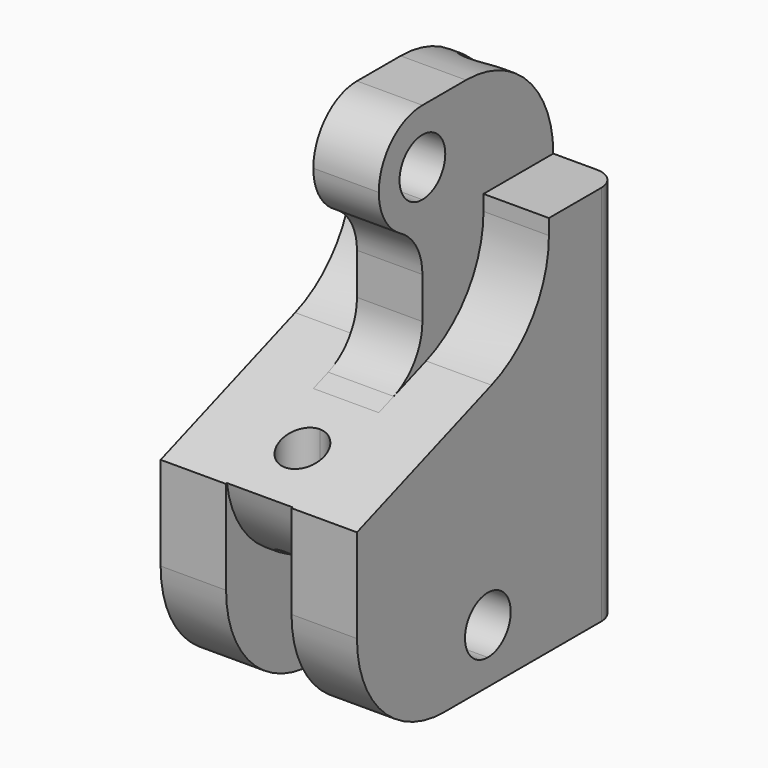
from build123d import *

# Parameters (mm, degrees)
F1_DEPTH     = 15
F3_DEPTH     = 6
F5_DEPTH     = 18
F6_R         = 10
F7_R         = 10
F10_DEPTH    = 6
F11_DEPTH    = 6
F12_R        = 2
F14_DEPTH    = 6
F18_DEPTH    = 40
F20_DEPTH    = 40
F22_DEPTH    = 6
F23_T1_DEPTH = 6


# Not quite as in the source:
# - a fillet or chamfer that OpenCascade refuses, or shapes differently, is made with other operations: its cross-section is extruded or revolved along the edge and cut away or added


with BuildPart() as f1:
    # F0 (on Front) → F1 (new body, symmetric)
    with BuildSketch(Plane.XZ):
        Polygon((9, -12.5), (9, 12.5), (3, 12.5), (3, 22.5), (-3, 22.5), (-3, 12.5), (-9, 12.5), (-9, -12.5), (-9, -22.5), (-3, -22.5), (-3, -12.5), (3, -12.5), (3, -22.5), (9, -22.5), align=None)
    extrude(amount=F1_DEPTH, both=True)

    # F2 (on face) → F3 (cut)
    with BuildSketch(Plane(origin=(-3, 0, 0), x_dir=(0, -1, 0), z_dir=(-1, 0, 0))):
        with BuildLine():
            ThreePointArc((0, 20.12), (-2.62, 17.5), (0, 14.88))
            Line((0, 14.88), (0, 20.12))
        make_face()
        with BuildLine():
            Line((0, 20.12), (0, 14.88))
            ThreePointArc((0, 14.88), (1.8526197667, 15.6473802333), (2.62, 17.5))
            ThreePointArc((2.62, 17.5), (1.8526197667, 19.3526197667), (0, 20.12))
        make_face()
    extrude(amount=-F3_DEPTH, mode=Mode.SUBTRACT)

    # F4 (on face) → F5 (cut)
    with BuildSketch(Plane(origin=(-9, 0, 0), x_dir=(0, -1, 0), z_dir=(-1, 0, 0))):
        with BuildLine():
            ThreePointArc((0, -20.12), (1.8526197667, -19.3526197667), (2.62, -17.5))
            ThreePointArc((2.62, -17.5), (-1.8526197667, -15.6473802333), (0, -20.12))
        make_face()
    extrude(amount=-F5_DEPTH, mode=Mode.SUBTRACT)

    # F6
    f6_edges = [f1.edges().sort_by_distance(p)[0] for p in [
        (0, -15, -12.5),
    ]]
    fillet(f6_edges, radius=F6_R)

    # F7
    f7_edges = [f1.edges().sort_by_distance(p)[0] for p in [
        (0, 15, 22.5),
        (0, -15, 22.5),
        (6, -15, -22.5),
        (-6, -15, -22.5),
    ]]
    fillet(f7_edges, radius=F7_R)

    # F9 (on face) → F10 (cut)
    with BuildSketch(Plane(origin=(-9, 0, 0), x_dir=(0, -1, 0), z_dir=(-1, 0, 0))):
        with BuildLine():
            ThreePointArc((-7, 11.0872004348), (-5.1915204429, 5.3514360713), (-0.4202014333, 1.690274227))
            Line((-0.4202014333, 1.690274227), (15, -3.9222201011))
            Line((15, -3.9222201011), (15, 12.5))
            Line((15, 12.5), (-7, 12.5))
            Line((-7, 12.5), (-7, 11.0872004348))
        make_face()
    extrude(amount=-F10_DEPTH, mode=Mode.SUBTRACT)

    # F8 (on face) → F11 (cut)
    with BuildSketch(Plane.YZ.offset(9)):
        with BuildLine():
            Line((7, 12.5), (-15, 12.5))
            Line((-15, 12.5), (-15, -3.92222))
            Line((-15, -3.92222), (0.4202014333, 1.6902743281))
            ThreePointArc((0.4202014333, 1.6902743281), (5.1915204429, 5.3514361724), (7, 11.087200536))
            Line((7, 11.087200536), (7, 12.5))
        make_face()
    extrude(amount=-F11_DEPTH, mode=Mode.SUBTRACT)

    # F12
    f12_edges = [f1.edges().sort_by_distance(p)[0] for p in [
        (9, 15, -5),
        (-9, 15, -5),
    ]]
    fillet(f12_edges, radius=F12_R)

    # F13 (on face) → F14 (cut)
    with BuildSketch(Plane(origin=(-3, 0, 0), x_dir=(0, -1, 0), z_dir=(-1, 0, 0))):
        with BuildLine():
            Line((5, 22.5), (0, 22.5))
            ThreePointArc((0, 22.5), (3.5355339059, 21.0355339059), (5, 17.5))
            Line((5, 17.5), (5, -0.2825177585))
            Line((5, -0.2825177585), (14.9033390576, -3.8870383953))
            ThreePointArc((14.9033390576, -3.8870383953), (14.9758054957, -3.1952012025), (15, -2.5))
            Line((15, -2.5), (15, 12.5))
            ThreePointArc((15, 12.5), (12.0710678119, 19.5710678119), (5, 22.5))
        make_face()
    extrude(amount=-F14_DEPTH, mode=Mode.SUBTRACT)

    # F17 (on face) → F18 (cut)
    with BuildSketch(Plane.XY.offset(17.5)):
        with BuildLine():
            ThreePointArc((2, -10), (1.4142135624, -8.5857864376), (0, -8))
            Line((0, -8), (0, -12))
            ThreePointArc((0, -12), (1.4142135624, -11.4142135624), (2, -10))
        make_face()
        with BuildLine():
            Line((0, -12), (0, -8))
            ThreePointArc((0, -8), (-2, -10), (0, -12))
        make_face()
    extrude(amount=-F18_DEPTH, mode=Mode.SUBTRACT)

    # F19 (on face) → F20 (cut)
    with BuildSketch(Plane(origin=(0, 0, -12.5), x_dir=(1, 0, 0), z_dir=(0, 0, -1))):
        with BuildLine():
            Line((0, -9), (0, -11))
            Line((0, -11), (0, -13))
            ThreePointArc((0, -13), (1.4142135624, -12.4142135624), (2, -11))
            ThreePointArc((2, -11), (1.4142135624, -9.5857864376), (0, -9))
        make_face()
        with BuildLine():
            Line((0, -13), (0, -11))
            Line((0, -11), (0, -9))
            ThreePointArc((0, -9), (-2, -11), (0, -13))
        make_face()
    extrude(amount=-F20_DEPTH, mode=Mode.SUBTRACT)

    # F21 (on face) → F22 (cut)
    with BuildSketch(Plane.YZ.offset(3)):
        with BuildLine():
            ThreePointArc((0, 12.5), (-3.5355339059, 13.9644660941), (-5, 17.5))
            Line((-5, 17.5), (-5, -0.2825177585))
            Line((-5.0000000325, -0.2825176692), (0, 1.537333514))
            Line((0, 1.537333514), (0, 12.5))
        make_face()
    extrude(amount=-F22_DEPTH, mode=Mode.SUBTRACT)

    # F23: fillet of radius 5 on 2 edges, made by hand

    # F23_s2 → F23_t1 (join)
    with BuildSketch(Plane.YZ.offset(-3)):
        with BuildLine():
            ThreePointArc((-2.5, 13.1698729811), (-0.6698729811, 11.3397459622), (0, 8.8397459622))
            Line((0, 8.8397459622), (0, 12.5))
            ThreePointArc((0, 12.5), (-1.2940952255, 12.6703708686), (-2.5, 13.1698729811))
        make_face()
        with BuildLine():
            ThreePointArc((0, 5.0383711039), (-0.9042397786, 2.1704889222), (-3.2898992834, 0.339908))
            Line((-3.2898992834, 0.339908), (0, 1.537333514))
            Line((0, 1.537333514), (0, 5.0383711039))
        make_face()
    extrude(amount=F23_T1_DEPTH)


solid = f1.part
